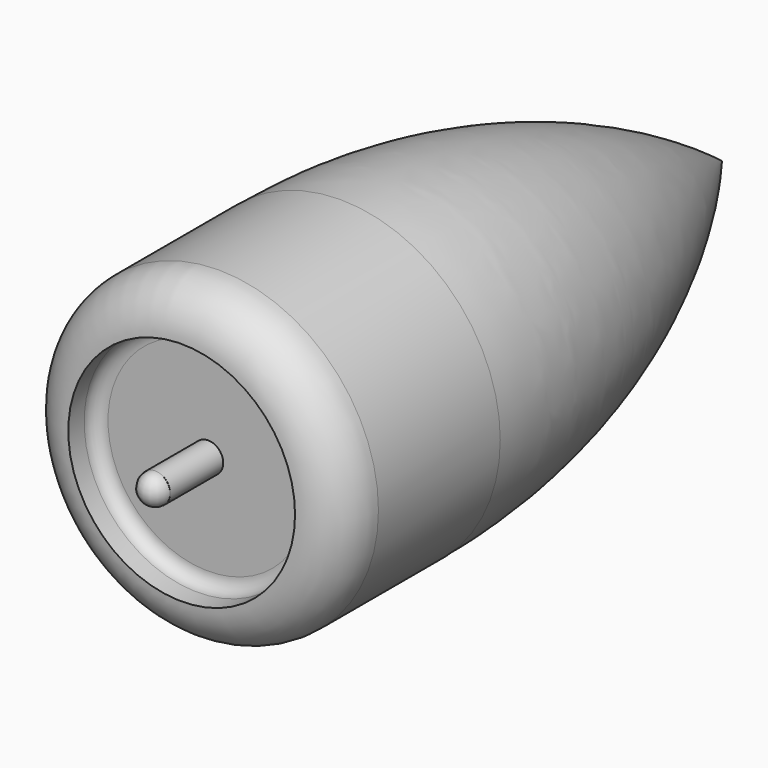
from build123d import *

# Parameters (mm, degrees)
F0_R     = 30.6426839296
F1_DEPTH = 38.1
F2_R     = 8.89
F3_DEPTH = 6.35
F4_R     = 2.8916869665
F5_DEPTH = 12.7
F10_R    = 2.54


with BuildPart() as f1:
    # F0 (on Front) → F1 (new body)
    with BuildSketch(Plane.XZ):
        Circle(F0_R)
    extrude(amount=F1_DEPTH)

    # F2
    f2_edges = [f1.edges().sort_by_distance(p)[0] for p in [
        (-30.642684, -38.1, 0),
    ]]
    fillet(f2_edges, radius=F2_R)

    # F3 (cut): a face of the model
    f3_faces = [f1.faces().sort_by_distance(p)[0] for p in [
        (0, -38.1, 0),
    ]]
    extrude(f3_faces, amount=-F3_DEPTH, mode=Mode.SUBTRACT)

    # F4 (on face) → F5 (join)
    with BuildSketch(Plane.XZ.offset(31.75)):
        Circle(F4_R)
    extrude(amount=F5_DEPTH)

    # F6 (on Right) → F7 (revolve)
    with BuildSketch(Plane.YZ):
        with BuildLine():
            Line((0, 30.5668525398), (0, 0))
            Line((0, 0), (91.4566889405, 0))
            ThreePointArc((91.4566889405, 0), (48.2448652239, 22.8129112072), (0, 30.5668525398))
        make_face()
    revolve(axis=Axis((0, 47.0633842051, 0), (0, -1, 0)))

    # F8 (on face) → F9 (revolve)
    with BuildSketch(Plane.XZ.offset(44.45)):
        with BuildLine():
            ThreePointArc((0, -2.8916869665), (2.8679164431, 0), (0, 2.8916869665))
            Line((0, 2.8916869665), (0, -2.8916869665))
        make_face()
    revolve(axis=Axis((0, -44.45, 0.0952386763), (0, 0, -1)))

    # F10
    f10_edges = [f1.edges().sort_by_distance(p)[0] for p in [
        (-21.752684, -31.75, 0),
    ]]
    fillet(f10_edges, radius=F10_R)


solid = f1.part
